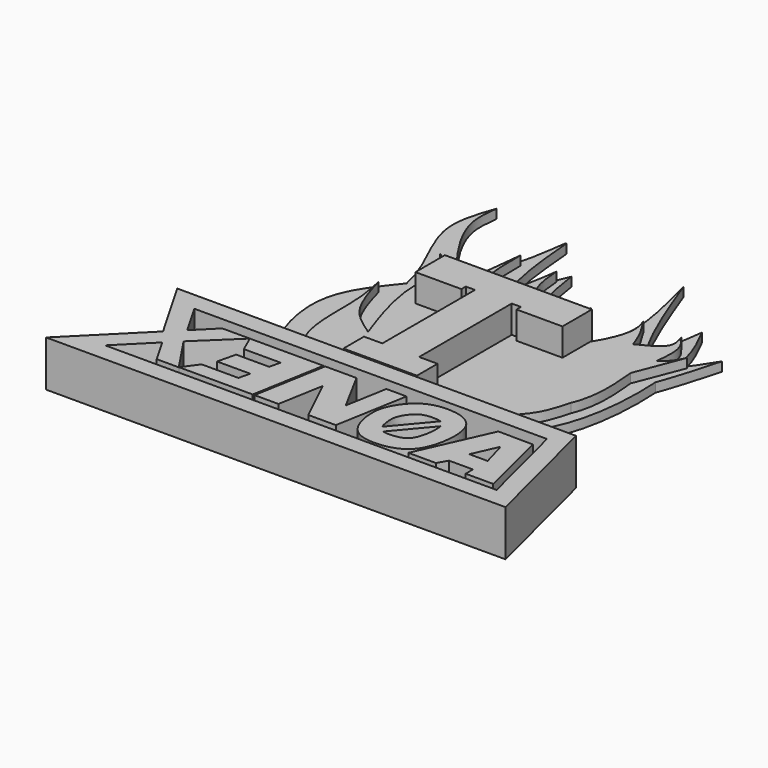
from build123d import *

# Parameters (mm, degrees)
F1_DEPTH = 25
F0_W     = 40
F0_H     = 1
F2_DEPTH = 20
F3_DEPTH = 5
F4_DEPTH = 5
F5_DEPTH = 5
F7_DEPTH = 5
F9_DEPTH = 5


# Not quite as in the source:
# - ends of sketch curves that miss each other by under 0.0002 mm in the source are joined
# - the dataset's text gives a spline's control points without its knots; the knots are read off the source's solid
# - a feature names something its author has since deleted; it is built from what else it names


with BuildPart() as f1:
    # F0 (on Top) → F1 (new body)
    with BuildSketch(Plane.XY):
        Polygon((35.3553390593, 35.3553390593), (0, 0), (250, 0), (232.3553390593, 69.9963552107), (145, 69.9963552107), (105, 69.9963552107), (15.3553390593, 69.9963552107), align=None)
        Polygon((32.6758509431, 59.9963530121), (224.56330661, 59.9963530121), (237.166372237, 10.0000021986), (24.1421409317, 10.0000021986), (41.4001874912, 27.2580487582), (47.8522307846, 33.7100920516), (42.6758487445, 42.6758487445), align=None, mode=Mode.SUBTRACT)
        Polygon((53.2824504623, 53.2824504623), (42.6758487445, 42.6758487445), (47.8522307846, 33.7100920516), (68.2824504623, 53.2824504623), align=None)
        Polygon((47.8522307846, 33.7100920516), (41.4001874912, 27.2580487582), (49.1933937334, 13.7598195929), (61.1933937334, 13.7598195929), align=None)
    extrude(amount=F1_DEPTH)


with BuildPart() as f1b:
    # F0 (on Top) → F1, piece 2 (new body)
    with BuildSketch(Plane.XY):
        Polygon((88.5540837341, 28.1308456181), (90.9036234209, 38.1308456181), (72.9036234209, 38.1308456181), (70.5540837341, 28.1308456181), align=None)
        Polygon((108.2824504623, 53.2824504623), (68.2824504623, 53.2824504623), (72.313347233, 44.1308456181), (92.313347233, 44.1308456181), (90.9036234209, 38.1308456181), (88.5540837341, 28.1308456181), (87.1034676285, 21.9568017674), (67.1034676285, 21.9568017674), (61.1933937334, 13.8901403418), (101.3365233556, 13.8901403418), align=None)
    extrude(amount=F1_DEPTH)


with BuildPart() as f1c:
    # F0 (on Top) → F1, piece 3 (new body)
    with BuildSketch(Plane.XY):
        Polygon((126.2824504623, 53.2824504623), (109.2824504623, 53.2824504623), (102.3365233556, 13.8901403418), (115.3365233556, 13.8901403418), (119.6777277973, 38.5103341671), (131.5355133201, 13.9200327762), (146.5355133201, 13.9200327762), (153.4814404268, 53.3123428967), (142.5191015005, 53.3123428967), (138.5251934142, 30.6617645774), align=None)
    extrude(amount=F1_DEPTH)


with BuildPart() as f1d:
    # F0 (on Top) → F1, piece 4 (new body)
    with BuildSketch(Plane.XY):
        with BuildLine():
            add(Edge.make_bspline(
                [(151.5315026045, 33.6161878365), (151.6881953051, 36.8603511522), (153.3257449913, 42.6794005447), (161.5552143615, 53.4867465492), (176.1548241084, 56.3217499328), (194.0088877696, 50.9134823684), (191.9976885112, 23.1984608195), (181.36266293, 11.4878216907), (160.3055787763, 10.4275817806), (152.5823075504, 20.9096175793), (151.3494491195, 29.8469552222), (151.5315026045, 33.6161878365)],
                knots=[0, 0, 0, 0, 0.0883183193, 0.1917010674, 0.3023367007, 0.4162516271, 0.5584218951, 0.6722296295, 0.7975352428, 0.8973873208, 1, 1, 1, 1], degree=3))
        make_face()
        with BuildLine():
            add(Edge.make_bspline(
                [(162.8184250503, 25.0692523461), (162.7388528349, 25.2709199434), (162.5250729743, 25.8491123795), (162.2111113791, 26.8772771924), (161.811446171, 28.5859325459), (161.5680124914, 30.3698864013), (161.490617043, 32.0313577817), (161.5032118997, 32.7877081125), (161.5198585813, 33.1337514359)],
                knots=[0.8971962129, 0.8971962129, 0.8971962129, 0.8971962129, 0.90625, 0.921875, 0.9375, 0.96875, 0.984375, 1, 1, 1, 1], degree=3))
            add(Edge.make_bspline(
                [(161.5198585813, 33.1337514359), (161.5365052629, 33.4797947593), (161.5904971328, 34.1076177221), (161.7198338174, 34.8971109654), (161.8983772283, 35.617959176), (162.1037900469, 36.2305480911), (162.3191108206, 36.7643620724), (162.5109148317, 37.1933987719), (162.7379267984, 37.6574642255), (163.0921353714, 38.326605495), (163.596210236, 39.1811127594), (164.287470415, 40.1970519056), (165.0414513207, 41.1551577869), (165.8327231283, 42.017135319), (166.4983498938, 42.6285934344), (167.0176778213, 43.0428000772), (167.3981141086, 43.3156806379), (167.7595288983, 43.5467960735), (168.1488651256, 43.766963423), (168.5654607343, 43.9738592368), (169.1603655772, 44.23185257), (169.9804869671, 44.5178805652), (171.0896341478, 44.7915612101), (172.3184150489, 44.9834054828), (173.6559028444, 45.0826399089), (174.7295299917, 45.0813201083), (175.4692709806, 45.0471315589), (175.9685909899, 45.0153875781), (176.5764482855, 44.960404607), (177.2752413398, 44.8700053931), (178.152789541, 44.7188709988), (178.7412145092, 44.5732668808), (179.0910574906, 44.4674492213), (179.0945257888, 44.4663980322)],
                knots=[0, 0, 0, 0, 0.015625, 0.03125, 0.046875, 0.0625, 0.0703125, 0.078125, 0.0859375, 0.09375, 0.109375, 0.125, 0.140625, 0.15625, 0.171875, 0.1796875, 0.1875, 0.1953125, 0.203125, 0.2109375, 0.21875, 0.234375, 0.25, 0.265625, 0.28125, 0.296875, 0.30078125, 0.3046875, 0.3125, 0.3203125, 0.328125, 0.34375, 0.3439066519, 0.3439066519, 0.3439066519, 0.3439066519], degree=3))
            add(Edge.make_bspline(
                [(179.0945257888, 44.4663980322), (179.4369974189, 44.3626000224), (180.0408289592, 44.137858269), (180.6603332198, 43.8043498556), (180.954614815, 43.5775919437), (181.1038370269, 43.4315691806), (181.1895827034, 43.3310307887), (181.2538264485, 43.2395291398), (181.3046724038, 43.1550069204), (181.3582155541, 43.05569095), (181.422796919, 42.9212624239), (181.5199173994, 42.6948431225), (181.7085595453, 42.1772024114), (181.8753089955, 41.5231873988), (181.9696544415, 41.0096622148), (181.9730783847, 40.9907957298)],
                knots=[0.3439066519, 0.3439066519, 0.3439066519, 0.3439066519, 0.359375, 0.375, 0.390625, 0.3984375, 0.40625, 0.4140625, 0.41796875, 0.421875, 0.42578125, 0.4296875, 0.4375, 0.453125, 0.4537178211, 0.4537178211, 0.4537178211, 0.4537178211], degree=3))
            add(Edge.make_bspline(
                [(181.9730783847, 40.9907957298), (182.0598994005, 40.512397778), (182.2045363428, 39.41183358), (182.2797979507, 37.4823107399), (182.193566141, 35.3678582229), (181.9493626032, 33.2017921364), (181.5644163989, 31.0887847577), (181.0667847965, 29.1323622869), (180.5011449009, 27.4494312491), (179.9317447836, 26.1476864655), (179.3824865747, 25.1785905134), (178.8685398921, 24.4779841747), (178.3709172748, 23.9520794031), (177.8264944089, 23.5060953751), (177.1374617731, 23.0738355235), (176.2112022482, 22.6358864412), (174.9558716393, 22.2007569681), (173.4559950281, 21.8323747048), (171.8198374216, 21.5722282716), (170.1442177268, 21.4412866926), (168.5280439261, 21.4466193999), (167.3160139795, 21.558065936), (166.4822451641, 21.6958640201), (166.0986472535, 21.7808626756), (165.9163137021, 21.8272428827), (165.8971010414, 21.8322026836)],
                knots=[0.4537178211, 0.4537178211, 0.4537178211, 0.4537178211, 0.46875, 0.484375, 0.5, 0.515625, 0.53125, 0.546875, 0.5625, 0.578125, 0.59375, 0.609375, 0.625, 0.640625, 0.65625, 0.671875, 0.6875, 0.703125, 0.71875, 0.734375, 0.75, 0.765625, 0.7734375, 0.78125, 0.7821827292, 0.7821827292, 0.7821827292, 0.7821827292], degree=3))
            add(Edge.make_bspline(
                [(165.8971010414, 21.8322026836), (165.7553892759, 21.868785963), (165.5531970067, 21.9272567748), (165.3254056153, 22.0041417656), (165.1739060305, 22.0612615773), (165.0494707627, 22.1134592968), (164.8977695401, 22.1837784003), (164.7376634219, 22.2699020236), (164.5740601511, 22.3743238889), (164.3757102389, 22.5229923761), (164.1329229874, 22.7478764528), (163.795317607, 23.1578632169), (163.4078371213, 23.7696356085), (163.0732924198, 24.4470716455), (162.8761783378, 24.9228825776), (162.8184250503, 25.0692523461)],
                knots=[0.7821827292, 0.7821827292, 0.7821827292, 0.7821827292, 0.7890625, 0.79296875, 0.796875, 0.80078125, 0.8046875, 0.8125, 0.8203125, 0.828125, 0.84375, 0.859375, 0.875, 0.890625, 0.8971962129, 0.8971962129, 0.8971962129, 0.8971962129], degree=3))
        make_face(mode=Mode.SUBTRACT)
        with BuildLine():
            add(Edge.make_bspline(
                [(179.0945257888, 44.4663980322), (179.4369974189, 44.3626000224), (180.0408289592, 44.137858269), (180.6603332198, 43.8043498556), (180.954614815, 43.5775919437), (181.1038370269, 43.4315691806), (181.1895827034, 43.3310307887), (181.2538264485, 43.2395291398), (181.3046724038, 43.1550069204), (181.3582155541, 43.05569095), (181.422796919, 42.9212624239), (181.5199173994, 42.6948431225), (181.7085595453, 42.1772024114), (181.8753089955, 41.5231873988), (181.9696544415, 41.0096622148), (181.9730783847, 40.9907957298)],
                knots=[0.3439066519, 0.3439066519, 0.3439066519, 0.3439066519, 0.359375, 0.375, 0.390625, 0.3984375, 0.40625, 0.4140625, 0.41796875, 0.421875, 0.42578125, 0.4296875, 0.4375, 0.453125, 0.4537178211, 0.4537178211, 0.4537178211, 0.4537178211], degree=3))
            Line((179.0945257888, 44.4663980322), (162.8183697977, 25.0692305451))
            add(Edge.make_bspline(
                [(165.8971010414, 21.8322026836), (165.7553892759, 21.868785963), (165.5531970067, 21.9272567748), (165.3254056153, 22.0041417656), (165.1739060305, 22.0612615773), (165.0494707627, 22.1134592968), (164.8977695401, 22.1837784003), (164.7376634219, 22.2699020236), (164.5740601511, 22.3743238889), (164.3757102389, 22.5229923761), (164.1329229874, 22.7478764528), (163.795317607, 23.1578632169), (163.4078371213, 23.7696356085), (163.0732924198, 24.4470716455), (162.8761783378, 24.9228825776), (162.8183697977, 25.0692305451)],
                knots=[0.7821827292, 0.7821827292, 0.7821827292, 0.7821827292, 0.7890625, 0.79296875, 0.796875, 0.80078125, 0.8046875, 0.8125, 0.8203125, 0.828125, 0.84375, 0.859375, 0.875, 0.890625, 0.8971962129, 0.8971962129, 0.8971962129, 0.8971962129], degree=3))
            Line((165.8971010414, 21.8322026836), (181.9730783847, 40.9907957298))
        make_face()
    extrude(amount=F1_DEPTH)


with BuildPart() as f1e:
    # F0 (on Top) → F1, piece 5 (new body)
    with BuildSketch(Plane.XY):
        Polygon((232.5355133201, 13.4541621667), (223.0829559751, 52.321232543), (204.0839364723, 52.5142556785), (186.5355133201, 13.258009744), (201.5355133201, 13.258009744), (204.5355133201, 18.4541621667), (217.5355133201, 18.4541621667), (217.5355133201, 13.4541621667), align=None)
        Polygon((213.6570562804, 42.148201446), (217.5355133201, 28.4541621667), (207.5355133201, 28.4541621667), align=None, mode=Mode.SUBTRACT)
    extrude(amount=F1_DEPTH)


with BuildPart() as f1f:
    # F0 (on Top) → F1, piece 6 (new body)
    with BuildSketch(Plane.XY):
        Polygon((115, 84.9963552107), (135, 84.9963552107), (135, 147.9963552107), (135, 164.9963552107), (115, 164.9963552107), (115, 147.9963552107), align=None)
        Polygon((110, 147.9963552107), (115, 147.9963552107), (115, 164.9963552107), (85, 164.9963552107), (85, 144.9963552107), (110, 144.9963552107), align=None)
        Polygon((135, 164.9963552107), (135, 147.9963552107), (140, 147.9963552107), (140, 144.9963552107), (165, 144.9963552107), (165, 164.9963552107), align=None)
        Polygon((105, 70.9963552107), (145, 70.9963552107), (145, 84.9963552107), (135, 84.9963552107), (115, 84.9963552107), (105, 84.9963552107), align=None)
    extrude(amount=F1_DEPTH)


with BuildPart() as f2:
    # F0 (on Top) → F2 (new body)
    with BuildSketch(Plane.XY):
        with Locations((125, 70.4963552107)):
            Rectangle(F0_W, F0_H)
    extrude(amount=F2_DEPTH)

    # F3 (cut): a face of the model
    f3_faces = [f2.faces().sort_by_distance(p)[0] for p in [
        (145, 70.4963552107, 10),
    ]]
    extrude(f3_faces, amount=-F3_DEPTH, mode=Mode.SUBTRACT)

    # F4 (cut): a face of the model
    f4_faces = [f2.faces().sort_by_distance(p)[0] for p in [
        (122.5, 70.4963552107, 0),
    ]]
    extrude(f4_faces, amount=-F4_DEPTH, mode=Mode.SUBTRACT)

    # F5 (cut): a face of the model
    f5_faces = [f2.faces().sort_by_distance(p)[0] for p in [
        (105, 70.4963552107, 12.5),
    ]]
    extrude(f5_faces, amount=-F5_DEPTH, mode=Mode.SUBTRACT)


with BuildPart() as f7:
    # F6 (on Top) → F7 (new body)
    with BuildSketch(Plane.XY):
        with BuildLine():
            add(Edge.make_bspline(
                [(72.6291313767, 64.4820928574), (67.8843899279, 69.0185368819), (55.8107699639, 80.5621165964), (36.8814669711, 129.9010723984), (56.629985978, 154.7833033859), (64.5461439533, 164.572704302)],
                knots=[0, 0, 0, 0, 0.101291346, 0.2577491799, 0.3512765265, 0.3512765265, 0.3512765265, 0.3512765265], degree=3))
            Line((72.6291313767, 64.4820928574), (151.0081738234, 67.9656043649))
            add(Edge.make_bspline(
                [(203.9840248557, 159.5166123049), (205.2502449986, 139.053075114), (200.9255720037, 87.8784136061), (168.0975879471, 74.7828315421), (151.0081738234, 67.9656043649)],
                knots=[0.3580997219, 0.3580997219, 0.3580997219, 0.3580997219, 0.6658430302, 1, 1, 1, 1], degree=3))
            add(Edge.make_bspline(
                [(203.9840248331, 159.516612308), (199.9318801691, 148.4778161664), (187.4526257463, 122.5507837592), (144.9689882527, 101.7211149237), (96.0167865606, 127.4147770624), (67.6941499114, 142.280548811)],
                knots=[0.1630556944, 0.1630556944, 0.1630556944, 0.1630556944, 0.3379625541, 0.6169601084, 1, 1, 1, 1], degree=3))
            add(Edge.make_bspline(
                [(67.6941499114, 142.280548811), (66.9326522518, 149.6794238076), (66.1711545922, 157.0782988042), (64.5461439533, 164.572704302)],
                knots=[0, 0, 0, 0, 0.2188354672, 0.2188354672, 0.2188354672, 0.2188354672], degree=3))
        make_face()
        with BuildLine():
            add(Edge.make_bspline(
                [(64.5461439533, 164.572704302), (63.6677051528, 168.6239864405), (59.105528765, 185.0817451309), (41.2816915568, 213.1642182092), (48.2453116697, 233.0326511082), (51.4377579093, 242.1412616968)],
                knots=[0.2188354672, 0.2188354672, 0.2188354672, 0.2188354672, 0.3371322713, 0.6961107077, 1, 1, 1, 1], degree=3))
            add(Edge.make_bspline(
                [(64.5461439533, 164.572704302), (69.1240877777, 170.2339515392), (73.8784841975, 176.055785513), (78.0120651576, 182.408011082)],
                knots=[0.3512765265, 0.3512765265, 0.3512765265, 0.3512765265, 0.4053637416, 0.4053637416, 0.4053637416, 0.4053637416], degree=3))
            add(Edge.make_bspline(
                [(51.4377579093, 242.1412616968), (50.7325629152, 236.7059121166), (49.0353056098, 223.6241590415), (62.2171007089, 201.3512643703), (74.3436575726, 185.993505274), (78.0120651576, 182.408011082)],
                knots=[0, 0, 0, 0, 0.186533273, 0.4489466926, 0.5605380749, 0.5605380749, 0.5605380749, 0.5605380749], degree=3))
        make_face()
        with BuildLine():
            add(Edge.make_bspline(
                [(64.5461439533, 164.572704302), (69.1240877777, 170.2339515392), (73.8784841975, 176.055785513), (78.0120651576, 182.408011082)],
                knots=[0.3512765265, 0.3512765265, 0.3512765265, 0.3512765265, 0.4053637416, 0.4053637416, 0.4053637416, 0.4053637416], degree=3))
            add(Edge.make_bspline(
                [(67.6941499114, 142.280548811), (66.9326522518, 149.6794238076), (66.1711545922, 157.0782988042), (64.5461439533, 164.572704302)],
                knots=[0, 0, 0, 0, 0.2188354672, 0.2188354672, 0.2188354672, 0.2188354672], degree=3))
            add(Edge.make_bspline(
                [(203.9840248331, 159.516612308), (199.9318801691, 148.4778161664), (187.4526257463, 122.5507837592), (144.9689882527, 101.7211149237), (96.0167865606, 127.4147770624), (67.6941499114, 142.280548811)],
                knots=[0.1630556944, 0.1630556944, 0.1630556944, 0.1630556944, 0.3379625541, 0.6169601084, 1, 1, 1, 1], degree=3))
            add(Edge.make_bspline(
                [(202.1716325366, 175.6673243605), (202.9959256883, 170.8074535364), (203.6245529634, 165.3260811228), (203.9840248557, 159.5166123049)],
                knots=[0.2707333426, 0.2707333426, 0.2707333426, 0.2707333426, 0.3580997219, 0.3580997219, 0.3580997219, 0.3580997219], degree=3))
            add(Edge.make_bspline(
                [(183.2629358632, 179.4378548769), (186.5818173417, 174.7291961232), (192.9735646115, 168.9927763491), (199.1793349579, 172.6329802706), (202.1716325366, 175.6673243605)],
                knots=[0.4351984528, 0.4351984528, 0.4351984528, 0.4351984528, 0.6115428484, 0.7784285065, 0.7784285065, 0.7784285065, 0.7784285065], degree=3))
            add(Edge.make_bspline(
                [(150.4996522715, 168.3783778708), (151.1264881336, 168.0576644253), (159.7492700166, 164.3286865117), (175.1084463246, 168.7794389692), (182.3271173997, 177.9847147478), (183.2629358632, 179.4378548769)],
                knots=[0.395429429, 0.395429429, 0.395429429, 0.395429429, 0.4182646932, 0.6968146028, 0.7451226477, 0.7451226477, 0.7451226477, 0.7451226477], degree=3))
            add(Edge.make_bspline(
                [(126.0291058523, 176.5534876593), (127.597006423, 174.4584276978), (133.9308745674, 168.2929781798), (144.0894313655, 166.9516503416), (150.4996522715, 168.3783778708)],
                knots=[0.2688699275, 0.2688699275, 0.2688699275, 0.2688699275, 0.3344549429, 0.4968084223, 0.4968084223, 0.4968084223, 0.4968084223], degree=3))
            add(Edge.make_bspline(
                [(103.0729814284, 186.3879106282), (104.479610769, 182.9302975439), (109.3195239872, 174.1790287586), (118.3190919374, 170.9636291209), (124.4153474267, 175.0946416403), (126.0291058523, 176.5534876593)],
                knots=[0.7654028494, 0.7654028494, 0.7654028494, 0.7654028494, 0.8060088233, 0.8849466927, 0.9139412888, 0.9139412888, 0.9139412888, 0.9139412888], degree=3))
            add(Edge.make_bspline(
                [(78.0120651576, 182.408011082), (82.5887153764, 177.9348023672), (91.8242455261, 172.1378203368), (99.4843649054, 180.4058618036), (103.0729814284, 186.3879106282)],
                knots=[0.5605380749, 0.5605380749, 0.5605380749, 0.5605380749, 0.6997578078, 0.8367611724, 0.8367611724, 0.8367611724, 0.8367611724], degree=3))
        make_face()
        with BuildLine():
            add(Edge.make_bspline(
                [(78.0120651576, 182.408011082), (80.3305164532, 185.9708602782), (92.2505240484, 206.9105530834), (94.34730672, 251.4608866795), (95.830261953, 215.4406179354), (99.9032976015, 194.1792597467), (103.0729814284, 186.3879106282)],
                knots=[0.4053637416, 0.4053637416, 0.4053637416, 0.4053637416, 0.4357002888, 0.5756823285, 0.6739017732, 0.7654028494, 0.7654028494, 0.7654028494, 0.7654028494], degree=3))
            add(Edge.make_bspline(
                [(78.0120651576, 182.408011082), (82.5887153764, 177.9348023672), (91.8242455261, 172.1378203368), (99.4843649054, 180.4058618036), (103.0729814284, 186.3879106282)],
                knots=[0.5605380749, 0.5605380749, 0.5605380749, 0.5605380749, 0.6997578078, 0.8367611724, 0.8367611724, 0.8367611724, 0.8367611724], degree=3))
        make_face()
        with BuildLine():
            add(Edge.make_bspline(
                [(202.1716325366, 175.6673243605), (202.9959256883, 170.8074535364), (203.6245529634, 165.3260811228), (203.9840248557, 159.5166123049)],
                knots=[0.2707333426, 0.2707333426, 0.2707333426, 0.2707333426, 0.3580997219, 0.3580997219, 0.3580997219, 0.3580997219], degree=3))
            add(Edge.make_bspline(
                [(214.0017002821, 192.2109127045), (210.8816542921, 181.0091826827), (207.7616083022, 169.8074526609), (203.9840248331, 159.516612308)],
                knots=[0, 0, 0, 0, 0.1630556944, 0.1630556944, 0.1630556944, 0.1630556944], degree=3))
            add(Edge.make_bspline(
                [(202.1716325366, 175.6673243605), (206.1444595091, 179.6959758322), (210.0730798956, 185.9534442683), (214.0017002821, 192.2109127045)],
                knots=[0.7784285065, 0.7784285065, 0.7784285065, 0.7784285065, 1, 1, 1, 1], degree=3))
        make_face()
        with BuildLine():
            add(Edge.make_bspline(
                [(103.0729814284, 186.3879106282), (107.3488001692, 193.5154920537), (111.3254802757, 203.3137369016), (115.3021603823, 213.1119817495)],
                knots=[0.8367611724, 0.8367611724, 0.8367611724, 0.8367611724, 1, 1, 1, 1], degree=3))
            add(Edge.make_bspline(
                [(103.0729814284, 186.3879106282), (104.479610769, 182.9302975439), (109.3195239872, 174.1790287586), (118.3190919374, 170.9636291209), (124.4153474267, 175.0946416403), (126.0291058523, 176.5534876593)],
                knots=[0.7654028494, 0.7654028494, 0.7654028494, 0.7654028494, 0.8060088233, 0.8849466927, 0.9139412888, 0.9139412888, 0.9139412888, 0.9139412888], degree=3))
            add(Edge.make_bspline(
                [(115.3021603823, 213.1119817495), (117.4517792341, 199.127150255), (119.601398086, 185.1423187605), (126.0291058523, 176.5534876593)],
                knots=[0, 0, 0, 0, 0.2688699275, 0.2688699275, 0.2688699275, 0.2688699275], degree=3))
        make_face()
        with BuildLine():
            add(Edge.make_bspline(
                [(183.2629358632, 179.4378548769), (186.5818173417, 174.7291961232), (192.9735646115, 168.9927763491), (199.1793349579, 172.6329802706), (202.1716325366, 175.6673243605)],
                knots=[0.4351984528, 0.4351984528, 0.4351984528, 0.4351984528, 0.6115428484, 0.7784285065, 0.7784285065, 0.7784285065, 0.7784285065], degree=3))
            add(Edge.make_bspline(
                [(190.778285265, 207.5964212418), (194.995258662, 199.5624456232), (199.4144388008, 191.143235411), (202.0547544684, 176.3564145378), (202.1716325366, 175.6673243605)],
                knots=[0, 0, 0, 0, 0.2583455002, 0.2707333426, 0.2707333426, 0.2707333426, 0.2707333426], degree=3))
            add(Edge.make_bspline(
                [(183.2629358632, 179.4378548769), (188.2003936461, 187.1047457544), (189.4893394555, 197.3505834981), (190.778285265, 207.5964212418)],
                knots=[0.7451226477, 0.7451226477, 0.7451226477, 0.7451226477, 1, 1, 1, 1], degree=3))
        make_face()
        with BuildLine():
            add(Edge.make_bspline(
                [(126.0291058523, 176.5534876593), (130.8188939141, 180.8834810058), (135.3979733609, 188.2889488836), (139.9770528078, 195.6944167614)],
                knots=[0.9139412888, 0.9139412888, 0.9139412888, 0.9139412888, 1, 1, 1, 1], degree=3))
            add(Edge.make_bspline(
                [(126.0291058523, 176.5534876593), (127.597006423, 174.4584276978), (133.9308745674, 168.2929781798), (144.0894313655, 166.9516503416), (150.4996522715, 168.3783778708)],
                knots=[0.2688699275, 0.2688699275, 0.2688699275, 0.2688699275, 0.3344549429, 0.4968084223, 0.4968084223, 0.4968084223, 0.4968084223], degree=3))
            add(Edge.make_bspline(
                [(139.9770528078, 195.6944167614), (139.3780866876, 191.5550232222), (138.1184145198, 182.8495578263), (144.8063069143, 171.2913133241), (150.4996522715, 168.3783778708)],
                knots=[0, 0, 0, 0, 0.1880241835, 0.395429429, 0.395429429, 0.395429429, 0.395429429], degree=3))
        make_face()
        with BuildLine():
            add(Edge.make_bspline(
                [(150.4996522715, 168.3783778708), (151.1264881336, 168.0576644253), (159.7492700166, 164.3286865117), (175.1084463246, 168.7794389692), (182.3271173997, 177.9847147478), (183.2629358632, 179.4378548769)],
                knots=[0.395429429, 0.395429429, 0.395429429, 0.395429429, 0.4182646932, 0.6968146028, 0.7451226477, 0.7451226477, 0.7451226477, 0.7451226477], degree=3))
            add(Edge.make_bspline(
                [(158.2654863596, 235.7548177242), (166.668895014, 213.4065606535), (175.0723036685, 191.0583035828), (183.2629358632, 179.4378548769)],
                knots=[0, 0, 0, 0, 0.4351984528, 0.4351984528, 0.4351984528, 0.4351984528], degree=3))
            add(Edge.make_bspline(
                [(150.4996522715, 168.3783778708), (154.9594308282, 169.3709940277), (173.0471745709, 178.929519006), (164.7219239532, 210.9343107789), (158.2654863596, 235.7548177242)],
                knots=[0.4968084223, 0.4968084223, 0.4968084223, 0.4968084223, 0.6097624963, 1, 1, 1, 1], degree=3))
        make_face()
    extrude(amount=F7_DEPTH)


with BuildPart() as f9:
    # F8 (on face) → F9 (new body)
    with BuildSketch(Plane.XY.offset(5)):
        with BuildLine():
            add(Edge.make_bspline(
                [(79.1123732924, 72.2368359566), (73.4663068627, 80.1369737675), (61.7622084436, 96.513683396), (64.430036356, 131.3518813145), (61.5910729249, 144.7565064772), (60.3671483696, 150.5354642868)],
                knots=[0, 0, 0, 0, 0.3464895496, 0.718260729, 1, 1, 1, 1], degree=3))
            add(Edge.make_bspline(
                [(193.6985125671, 114.7679910064), (187.7127476331, 100.4195530427), (155.272743548, 70.3517997269), (106.0212606403, 71.5708172991), (79.1123732924, 72.2368359566)],
                knots=[0.2773217653, 0.2773217653, 0.2773217653, 0.2773217653, 0.6051597625, 1, 1, 1, 1], degree=3))
            add(Edge.make_bspline(
                [(196.3944137096, 152.1943211555), (197.5781753136, 139.5499067734), (198.7619369175, 126.9054923913), (193.6985125671, 114.7679910064)],
                knots=[0, 0, 0, 0, 0.2773217653, 0.2773217653, 0.2773217653, 0.2773217653], degree=3))
            add(Edge.make_bspline(
                [(198.0532854795, 167.4559265375), (200.1856301699, 169.1749374439), (203.9720421348, 172.2273911551), (208.648961946, 183.5796146754), (201.440390323, 165.117641873), (196.3944137096, 152.1943211555)],
                knots=[0, 0, 0, 0, 0.2788894417, 0.4952249623, 1, 1, 1, 1], degree=3))
            add(Edge.make_bspline(
                [(192.744910717, 191.1777555943), (194.9151137959, 188.5270944195), (199.7062970058, 182.6751981434), (198.6377990915, 172.837541412), (198.0532854795, 167.4559265375)],
                knots=[0, 0, 0, 0, 0.4529576482, 1, 1, 1, 1], degree=3))
            add(Edge.make_bspline(
                [(180.6351542473, 173.427850008), (186.1932461693, 176.1636989449), (195.9227247039, 180.9528215212), (193.6985125671, 188.1094463448), (192.744910717, 191.1777555943)],
                knots=[0, 0, 0, 0, 0.5712630849, 1, 1, 1, 1], degree=3))
            add(Edge.make_bspline(
                [(170.681938529, 193.168386817), (172.9748754659, 189.5306996311), (177.289351154, 182.6858917028), (179.5676581625, 176.3816769328), (180.6351542473, 173.427850008)],
                knots=[0, 0, 0, 0, 0.5314520472, 1, 1, 1, 1], degree=3))
            add(Edge.make_bspline(
                [(131.6985189915, 176.5534876593), (131.5038840944, 174.2837643292), (130.9775051664, 168.1454276209), (152.4111091969, 139.8959369542), (175.6638281993, 179.9820987229), (172.0736437987, 189.4847591489), (170.681938529, 193.168386817)],
                knots=[0, 0, 0, 0, 0.1660205245, 0.4489929968, 0.7864066955, 1, 1, 1, 1], degree=3))
            add(Edge.make_bspline(
                [(123.9018365741, 170.2125880498), (126.5007307132, 172.3262212529), (129.0996248523, 174.4398544561), (131.6985189915, 176.5534876593)],
                knots=[0, 0, 0, 0, 10.0496400222, 10.0496400222, 10.0496400222, 10.0496400222], degree=3))
            add(Edge.make_bspline(
                [(113.4509593248, 205.2781432867), (113.7341524424, 201.0849296316), (114.3918216795, 191.3468835609), (120.4514761653, 177.8803927069), (123.9018365741, 170.2125880498)],
                knots=[0, 0, 0, 0, 0.4306011313, 1, 1, 1, 1], degree=3))
            add(Edge.make_bspline(
                [(106.3178256154, 167.4559265375), (108.6205358137, 178.350072301), (112.2154037568, 195.3574297189), (113.1242713149, 202.6550494687), (113.4509593248, 205.2781432867)],
                knots=[0, 0, 0, 0, 0.6405548784, 1, 1, 1, 1], degree=3))
            add(Edge.make_bspline(
                [(92.217437923, 207.2687745094), (92.1744035, 196.05093561), (92.100691159, 176.8362439496), (102.1397338037, 170.2125880498), (106.3178256154, 167.4559265375)],
                knots=[0, 0, 0, 0, 0.5838157124, 1, 1, 1, 1], degree=3))
            add(Edge.make_bspline(
                [(85.5819582939, 155.1802903414), (87.4838810338, 168.7831747375), (90.6082243427, 191.1290250462), (91.7648861314, 202.7298664214), (92.217437923, 207.2687745094)],
                knots=[0, 0, 0, 0, 0.6087431988, 1, 1, 1, 1], degree=3))
            add(Edge.make_bspline(
                [(64.5461439533, 187.3623579741), (69.0761925948, 184.3909963696), (79.0085918984, 177.8761104893), (83.2661963559, 163.1759067863), (85.5819582939, 155.1802903414)],
                knots=[0, 0, 0, 0, 0.4560880511, 1, 1, 1, 1], degree=3))
            add(Edge.make_bspline(
                [(85.5819582939, 112.0496988297), (80.9772279974, 125.1897638075), (72.693253835, 148.8289243578), (75.4374109757, 176.2326325502), (67.7985477289, 184.0387445767), (64.5461439533, 187.3623579741)],
                knots=[0, 0, 0, 0, 0.4181555726, 0.7522677195, 1, 1, 1, 1], degree=3))
            add(Edge.make_bspline(
                [(60.3671483696, 150.5354642868), (62.9949053402, 141.2496361384), (67.8923961206, 123.9431430899), (79.9799854745, 115.8161431782), (85.5819582939, 112.0496988297)],
                knots=[0, 0, 0, 0, 0.5365516932, 1, 1, 1, 1], degree=3))
        make_face()
        with BuildLine():
            add(Edge.make_bspline(
                [(193.6985125671, 114.7679910064), (187.7127476331, 100.4195530427), (155.272743548, 70.3517997269), (106.0212606403, 71.5708172991), (79.1123732924, 72.2368359566)],
                knots=[0.2773217653, 0.2773217653, 0.2773217653, 0.2773217653, 0.6051597625, 1, 1, 1, 1], degree=3))
            Line((79.1123732924, 72.2368359566), (81.4625397325, 68.5900822282))
            Line((81.4625397325, 68.5900822282), (140.8868581057, 67.9623708129))
            add(Edge.make_bspline(
                [(140.8868581057, 67.9623708129), (149.7084766463, 71.3167777423), (167.1102560461, 77.9337776877), (188.7068876338, 96.1144480526), (192.1413933904, 108.949086374), (193.6985125671, 114.7679910064)],
                knots=[0, 0, 0, 0, 0.359798311, 0.7097485351, 1, 1, 1, 1], degree=3))
        make_face()
    extrude(amount=F9_DEPTH)


solid = Compound([f1.part, f1b.part, f1c.part, f1d.part, f1e.part, f1f.part, f2.part, f7.part, f9.part])
